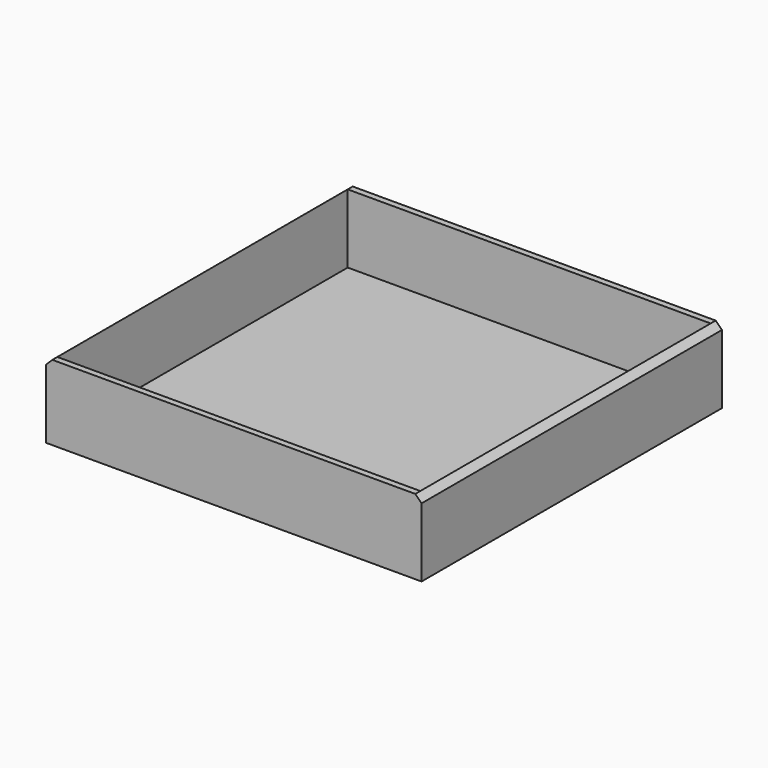
from build123d import *

# Parameters (mm, degrees)
F0_W     = 76.2
F0_H     = 76.2
F0_W_2   = 73.66
F0_H_2   = 73.66
F1_DEPTH = 13.97
F2_SIZE  = 1.26999
F3_W     = 76.2
F3_H     = 76.2
F4_DEPTH = 1.27


# Not quite as in the source:
# - a fillet or chamfer is up to 0.001 mm smaller than in the source, because OpenCascade refuses the exact size


with BuildPart() as f1:
    # F0 (on Top) → F1 (new body)
    with BuildSketch(Plane.XY):
        Rectangle(F0_W, F0_H)
        Rectangle(F0_W_2, F0_H_2, mode=Mode.SUBTRACT)
    extrude(amount=F1_DEPTH)

    # F2 (size 1.27 in the source; OpenCascade refuses exactly that, so slightly less here)
    f2_edges = [f1.edges().sort_by_distance(p)[0] for p in [
        (-38.1, 0, 13.97),
        (38.1, 0, 13.97),
    ]]
    chamfer(f2_edges, length=F2_SIZE)

    # F3 (on face) → F4 (join)
    with BuildSketch(Plane(origin=(0, 0, 0), x_dir=(1, 0, 0), z_dir=(0, 0, -1))):
        Rectangle(F3_W, F3_H)
    extrude(amount=F4_DEPTH)


solid = f1.part
